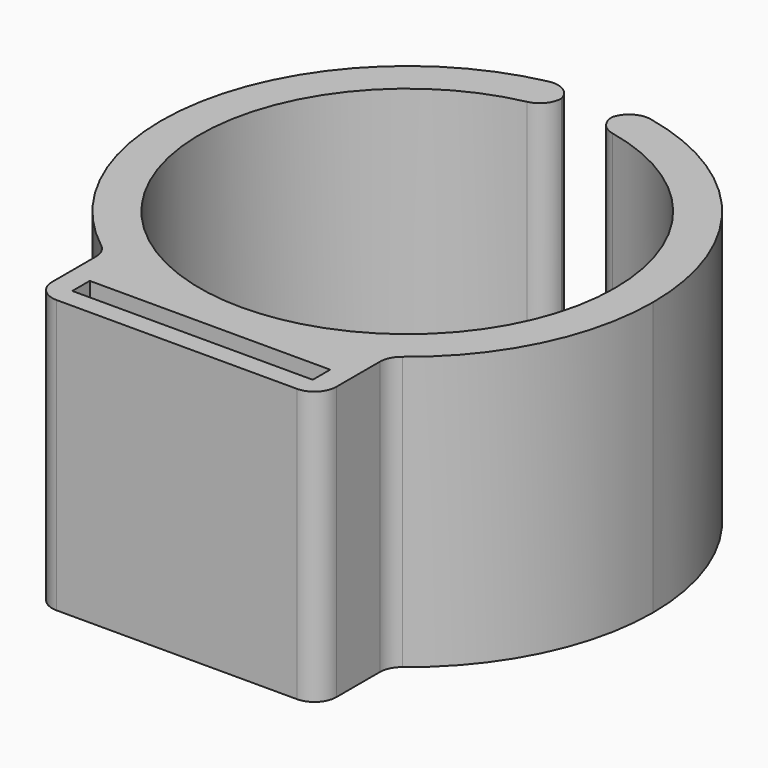
from build123d import *

# Parameters (mm, degrees)
F0_W        = 22
F0_H        = 2
F1_DEPTH    = 25
F2_T1_DEPTH = 25
F2_T3_DEPTH = 35.98872287
F2_T5_DEPTH = 34.5227248018
F2_T7_DEPTH = 35


# Not quite as in the source:
# - a fillet or chamfer that OpenCascade refuses, or shapes differently, is made with other operations: its cross-section is extruded or revolved along the edge and cut away or added


with BuildPart() as f1:
    # F0 (on Top) → F1 (new body)
    with BuildSketch(Plane.XY):
        with BuildLine():
            ThreePointArc((-4.8733971724, -18.3643676722), (-18.9479647202, 1.4052163402), (-2.1111111111, 18.88235181))
            Line((-2.1111111111, 18.88235181), (-2.5, 22.360679775))
            ThreePointArc((-2.5, 22.360679775), (-21.7874934858, 5.6173950908), (-13, -18.3643676722))
            Line((-13, -18.3643676722), (-4.8733971724, -18.3643676722))
        make_face()
        with BuildLine():
            ThreePointArc((2.1111111111, 18.88235181), (14.1617638575, 12.6666666667), (19, 0))
            ThreePointArc((19, 0), (15.0597899434, -11.5845900602), (4.8733971724, -18.3643676722))
            Line((4.8733971724, -18.3643676722), (13, -18.3643676722))
            ThreePointArc((13, -18.3643676722), (19.9843688917, -10.3380365641), (22.5, 0))
            ThreePointArc((22.5, 0), (16.7705098312, 15), (2.5, 22.360679775))
            Line((2.5, 22.360679775), (2.1111111111, 18.88235181))
        make_face()
        with BuildLine():
            Line((13, -18.3643676722), (4.8733971724, -18.3643676722))
            ThreePointArc((4.8733971724, -18.3643676722), (0, -19), (-4.8733971724, -18.3643676722))
            Line((-4.8733971724, -18.3643676722), (-13, -18.3643676722))
            ThreePointArc((-13, -18.3643676722), (0, -22.5), (13, -18.3643676722))
        make_face()
        with BuildLine():
            Line((13, -26.3643676722), (13, -18.3643676722))
            ThreePointArc((13, -18.3643676722), (0, -22.5), (-13, -18.3643676722))
            Line((-13, -18.3643676722), (-13, -26.3643676722))
            Line((-13, -26.3643676722), (13, -26.3643676722))
        make_face()
        with Locations((0, -23.5643676722)):
            Rectangle(F0_W, F0_H, mode=Mode.SUBTRACT)
    extrude(amount=F1_DEPTH)

    # F2: fillet of radius 2 on 8 edges, made by hand

    # F2_s2 → F2_t1 (join)
    with BuildSketch(Plane.XY):
        with BuildLine():
            ThreePointArc((-13.7755102041, -17.79003425), (-13.2043135586, -18.490740056), (-13, -19.3713706278))
            Line((-13, -19.3713706278), (-13, -18.3643676722))
            ThreePointArc((-13, -18.3643676722), (-13.390834604, -18.0813591471), (-13.7755102041, -17.79003425))
        make_face()
        with BuildLine():
            ThreePointArc((13, -19.3713706278), (13.2043135586, -18.490740056), (13.7755102041, -17.79003425))
            ThreePointArc((13.7755102041, -17.79003425), (13.390834604, -18.0813591471), (13, -18.3643676722))
            Line((13, -18.3643676722), (13, -19.3713706278))
        make_face()
    extrude(amount=F2_T1_DEPTH)

    # F2_s4 → F2_t3 (cut)
    with BuildSketch(Plane.XY.offset(-5.494361435)):
        with BuildLine():
            ThreePointArc((-2.2669117515, 20.275875101), (-3.0840105352, 21.6753462818), (-4.6696036077, 22.0101068182))
            ThreePointArc((-4.6696036077, 22.0101068182), (-3.5890847472, 22.2118993037), (-2.5, 22.360679775))
            Line((-2.5, 22.360679775), (-2.2669117515, 20.275875101))
        make_face()
        with BuildLine():
            ThreePointArc((2.2669117515, 20.275875101), (3.0840105352, 21.6753462818), (4.6696036077, 22.0101068182))
            ThreePointArc((4.6696036077, 22.0101068182), (3.5890847472, 22.2118993037), (2.5, 22.360679775))
            Line((2.5, 22.360679775), (2.2669117515, 20.275875101))
        make_face()
    extrude(amount=F2_T3_DEPTH, mode=Mode.SUBTRACT)

    # F2_s6 → F2_t5 (cut)
    with BuildSketch(Plane.XY.offset(-4.7613624009)):
        with BuildLine():
            ThreePointArc((-2.3227272178, 20.7751038089), (-2.6900167457, 19.3804728744), (-3.8998343218, 18.5954642927))
            ThreePointArc((-3.8998343218, 18.5954642927), (-3.0088938767, 18.7602387415), (-2.1111111111, 18.88235181))
            Line((-2.1111111111, 18.88235181), (-2.3227272178, 20.7751038089))
        make_face()
        with BuildLine():
            ThreePointArc((3.8998343218, 18.5954642927), (2.6900167457, 19.3804728744), (2.3227272178, 20.7751038089))
            Line((2.3227272178, 20.7751038089), (2.1111111111, 18.88235181))
            ThreePointArc((2.1111111111, 18.88235181), (3.0088938767, 18.7602387415), (3.8998343218, 18.5954642927))
        make_face()
    extrude(amount=F2_T5_DEPTH, mode=Mode.SUBTRACT)

    # F2_s8 → F2_t7 (cut)
    with BuildSketch(Plane.XY.offset(-5)):
        with BuildLine():
            ThreePointArc((11, -26.3643676722), (12.4142135624, -25.7785812346), (13, -24.3643676722))
            Line((13, -24.3643676722), (13, -26.3643676722))
            Line((13, -26.3643676722), (11, -26.3643676722))
        make_face()
        with BuildLine():
            ThreePointArc((-13, -24.3643676722), (-12.4142135624, -25.7785812346), (-11, -26.3643676722))
            Line((-11, -26.3643676722), (-13, -26.3643676722))
            Line((-13, -26.3643676722), (-13, -24.3643676722))
        make_face()
    extrude(amount=F2_T7_DEPTH, mode=Mode.SUBTRACT)


solid = f1.part
